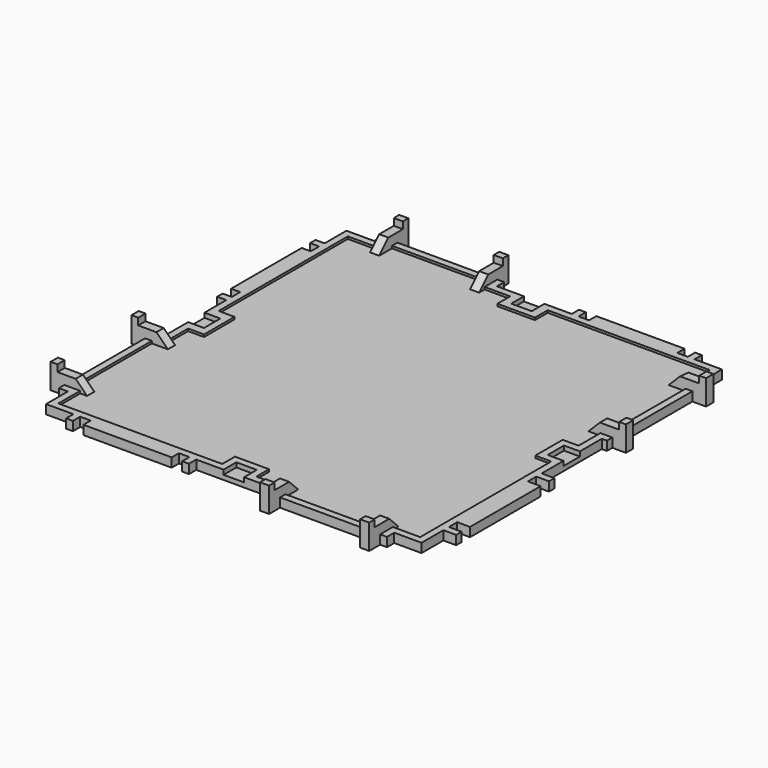
from build123d import *

# Parameters (mm, degrees)
F1_DEPTH = 3
F0_W     = 39.9216501117
F0_H     = 3
F0_W_2   = 3
F0_H_2   = 40
F0_W_3   = 40
F0_H_3   = 40.3722185198
F2_DEPTH = 4
F0_W_4   = 7
F0_H_4   = 9
F0_W_5   = 9
F0_H_5   = 7
F3_DEPTH = 2
F4_DEPTH = 8
F0_H_6   = 4
F0_W_6   = 4
F5_DEPTH = 11
F6_SIZE  = 4.99999


# Not quite as in the source:
# - a fillet or chamfer is up to 0.001 mm smaller than in the source, because OpenCascade refuses the exact size


with BuildPart() as f1:
    # F0 (on Top) → F1 (new body)
    with BuildSketch(Plane.XY):
        Polygon((-71.7994198203, 65.224928081), (-71.7994198203, 68.224928081), (-84, 68.224928081), (-84, -2.7506086044), (-77, -2.7506086044), (-77, -19.5105448365), (-84, -19.5105448365), (-84, -30.4028533991), (-81, -30.4028533991), (-81, -34.4028533991), (-88, -34.4028533991), (-88, -74.775071919), (-81, -74.775071919), (-81, -78.775071919), (-84, -78.775071919), (-84, -90.775071919), (-12, -90.775071919), (-12, -83.775071919), (3, -83.775071919), (3, -90.775071919), (15, -90.775071919), (15, -87.775071919), (19, -87.775071919), (19, -94.775071919), (59, -94.775071919), (59, -87.775071919), (63, -87.775071919), (63, -90.775071919), (75, -90.775071919), (75, -18.775071919), (68.6397999525, -18.775071919), (68, -18.775071919), (68, -3.775071919), (75, -3.775071919), (75, 8.224928081), (69.781611979, 8.224928081), (69.781611979, 12.224928081), (77.218388021, 12.224928081), (77.218388021, 52.224928081), (69.781611979, 52.224928081), (70.218388021, 56.224928081), (75, 56.224928081), (75, 68.224928081), (3.8335430436, 68.224928081), (3.8335430436, 61.224928081), (-12.6577513292, 61.224928081), (-12.6577513292, 68.224928081), (-23.8777697086, 68.224928081), (-23.8777697086, 65.224928081), (-27.8777697086, 65.224928081), (-27.8777697086, 72.224928081), (-67.7994198203, 72.224928081), (-67.7994198203, 65.224928081), align=None)
    extrude(amount=F1_DEPTH)

    # F0 (on Top) → F2 (join)
    with BuildSketch(Plane.XY):
        Polygon((-74.8768895864, 71.224928081), (-87, 71.224928081), (-87, 59.224928081), (-91, 59.224928081), (-91, 56.224928081), (-87, 56.224928081), (-87, 51.624928081), (-91, 51.624928081), (-91, 12.824928081), (-87, 12.824928081), (-87, 8.224928081), (-91, 8.224928081), (-91, 5.224928081), (-87, 5.224928081), (-87, -6.775071919), (-80, -6.775071919), (-80, -15.775071919), (-87, -15.775071919), (-87, -27.4028533991), (-91, -27.4028533991), (-91, -30.4028533991), (-84, -30.4028533991), (-84, -19.5105448365), (-77, -19.5105448365), (-77, -2.7506086044), (-84, -2.7506086044), (-84, 68.224928081), (-71.7994198203, 68.224928081), (-71.7994198203, 75.224928081), (-74.8768895864, 75.224928081), align=None)
        with Locations((-47.8385947645, 73.724928081)):
            Rectangle(F0_W, F0_H)
        Polygon((-20.8768895864, 75.224928081), (-23.8777697086, 75.224928081), (-23.8777697086, 68.224928081), (-12.6577513292, 68.224928081), (-12.6577513292, 61.224928081), (3.8335430436, 61.224928081), (3.8335430436, 68.224928081), (75, 68.224928081), (75, 56.224928081), (80.218388021, 56.224928081), (80.218388021, 59.224928081), (78, 59.224928081), (78, 71.224928081), (66, 71.224928081), (66, 75.224928081), (62.9867989421, 75.224928081), (63, 71.224928081), (58.4, 71.224928081), (58.3867989421, 75.224928081), (19.6, 75.224928081), (19.6, 71.224928081), (15, 71.224928081), (15, 75.224928081), (12, 75.224928081), (12, 71.224928081), (0, 71.224928081), (0, 64.224928081), (-9, 64.224928081), (-9, 71.224928081), (-20.8768895864, 71.224928081), align=None)
        with Locations((78.718388021, 32.224928081)):
            Rectangle(F0_W_2, F0_H_2)
        Polygon((79.781611979, 8.224928081), (75, 8.224928081), (75, -3.775071919), (68, -3.775071919), (68, -18.775071919), (68.6397999525, -18.775071919), (75, -18.775071919), (75, -90.775071919), (63, -90.775071919), (63, -97.775071919), (66, -97.775071919), (66, -93.775071919), (78, -93.775071919), (78, -81.775071919), (83.6185051799, -81.775071919), (83.6185051799, -78.775071919), (78, -78.775071919), (78, -74.175071919), (83.6185051799, -74.175071919), (83.6185051799, -35.375071919), (78, -35.375071919), (78, -30.775071919), (83.6185051799, -30.775071919), (83.6185051799, -27.775071919), (78, -27.775071919), (78, -15.775071919), (71, -15.775071919), (71, -6.775071919), (78, -6.775071919), (78, 5.224928081), (80.218388021, 5.224928081), (80.218388021, 8.224928081), align=None)
        with Locations((39, -96.275071919)):
            Rectangle(F0_W_3, F0_H)
        Polygon((-84, -90.775071919), (-84, -78.775071919), (-91, -78.775071919), (-91, -81.775071919), (-87, -81.775071919), (-87, -93.775071919), (-75, -93.775071919), (-75, -97.775071919), (-72, -97.775071919), (-72, -93.775071919), (-67.4, -93.775071919), (-67.4, -97.775071919), (-28.6, -97.775071919), (-28.6, -93.775071919), (-24, -93.775071919), (-24, -97.775071919), (-21, -97.775071919), (-21, -93.775071919), (-9, -93.775071919), (-9, -86.775071919), (0, -86.775071919), (0, -93.775071919), (12, -93.775071919), (12, -97.775071919), (15, -97.775071919), (15, -97.4028533991), (15, -90.775071919), (3, -90.775071919), (3, -83.775071919), (-12, -83.775071919), (-12, -90.775071919), align=None)
        with Locations((-89.5, -54.5889626591)):
            Rectangle(F0_W_2, F0_H_3)
    extrude(amount=F2_DEPTH)

    # F0 (on Top) → F3 (join)
    with BuildSketch(Plane.XY):
        with Locations((-83.5, -11.275071919)):
            Rectangle(F0_W_4, F0_H_4)
        with Locations((-4.5, 67.724928081)):
            Rectangle(F0_W_5, F0_H_5)
        with Locations((74.5, -11.275071919)):
            Rectangle(F0_W_4, F0_H_4)
        with Locations((-4.5, -90.275071919)):
            Rectangle(F0_W_5, F0_H_5)
    extrude(amount=F3_DEPTH)

    # F0 (on Top) → F4 (join)
    with BuildSketch(Plane.XY):
        Polygon((-71.7994198203, 78.224928081), (-71.7994198203, 75.224928081), (-71.7994198203, 68.224928081), (-71.7994198203, 65.224928081), (-67.7994198203, 65.224928081), (-67.7994198203, 72.224928081), (-67.7994198203, 75.224928081), (-67.7994198203, 78.224928081), align=None)
        Polygon((-27.8777697086, 78.224928081), (-27.8777697086, 75.224928081), (-27.8777697086, 72.224928081), (-27.8777697086, 65.224928081), (-23.8777697086, 65.224928081), (-23.8777697086, 68.224928081), (-23.8777697086, 75.224928081), (-23.8777697086, 78.224928081), align=None)
        Polygon((80.218388021, 56.224928081), (75, 56.224928081), (70.218388021, 56.224928081), (69.781611979, 52.224928081), (77.218388021, 52.224928081), (80.218388021, 52.224928081), (83.218388021, 52.224928081), (83.218388021, 56.224928081), align=None)
        Polygon((80.218388021, 12.224928081), (77.218388021, 12.224928081), (69.781611979, 12.224928081), (69.781611979, 8.224928081), (75, 8.224928081), (79.781611979, 8.224928081), (80.218388021, 8.224928081), (83.218388021, 8.224928081), (83.218388021, 12.224928081), align=None)
        Polygon((59, -87.775071919), (59, -94.775071919), (59, -97.775071919), (59, -100.775071919), (63, -100.775071919), (63, -97.775071919), (63, -90.775071919), (63, -87.775071919), align=None)
        Polygon((15, -87.775071919), (15, -90.775071919), (15, -97.4028533991), (15, -97.775071919), (15, -100.775071919), (19, -100.775071919), (19, -97.775071919), (19, -94.775071919), (19, -87.775071919), align=None)
        Polygon((-81, -30.4028533991), (-84, -30.4028533991), (-91, -30.4028533991), (-94, -30.4028533991), (-94, -34.4028533991), (-91, -34.4028533991), (-88, -34.4028533991), (-81, -34.4028533991), align=None)
        Polygon((-81, -74.775071919), (-88, -74.775071919), (-91, -74.775071919), (-91.2415088892, -74.775071919), (-94, -74.775071919), (-94, -78.775071919), (-91, -78.775071919), (-84, -78.775071919), (-81, -78.775071919), align=None)
    extrude(amount=F4_DEPTH)

    # F0 (on Top) → F5 (join)
    with BuildSketch(Plane.XY):
        with Locations((-95.5, -32.4028533991)):
            Rectangle(F0_W_2, F0_H_6)
        with Locations((-95.5, -76.775071919)):
            Rectangle(F0_W_2, F0_H_6)
        with Locations((17, -102.275071919)):
            Rectangle(F0_W_6, F0_H)
        with Locations((61, -102.275071919)):
            Rectangle(F0_W_6, F0_H)
        with Locations((84.718388021, 10.224928081)):
            Rectangle(F0_W_2, F0_H_6)
        with Locations((84.718388021, 54.224928081)):
            Rectangle(F0_W_2, F0_H_6)
        with Locations((-25.8777697086, 79.724928081)):
            Rectangle(F0_W_6, F0_H)
        with Locations((-69.7994198203, 79.724928081)):
            Rectangle(F0_W_6, F0_H)
    extrude(amount=F5_DEPTH)

    # F6 (size 5 in the source; OpenCascade refuses exactly that, so slightly less here)
    f6_edges = [f1.edges().sort_by_distance(p)[0] for p in [
        (-69.79942, 65.224928, 8),
        (-25.87777, 65.224928, 8),
        (70, 54.224928, 8),
        (69.781612, 10.224928, 8),
        (-81, -76.775072, 8),
        (-81, -32.402853, 8),
        (61, -87.775072, 8),
        (17, -87.775072, 8),
    ]]
    chamfer(f6_edges, length=F6_SIZE)


solid = f1.part
